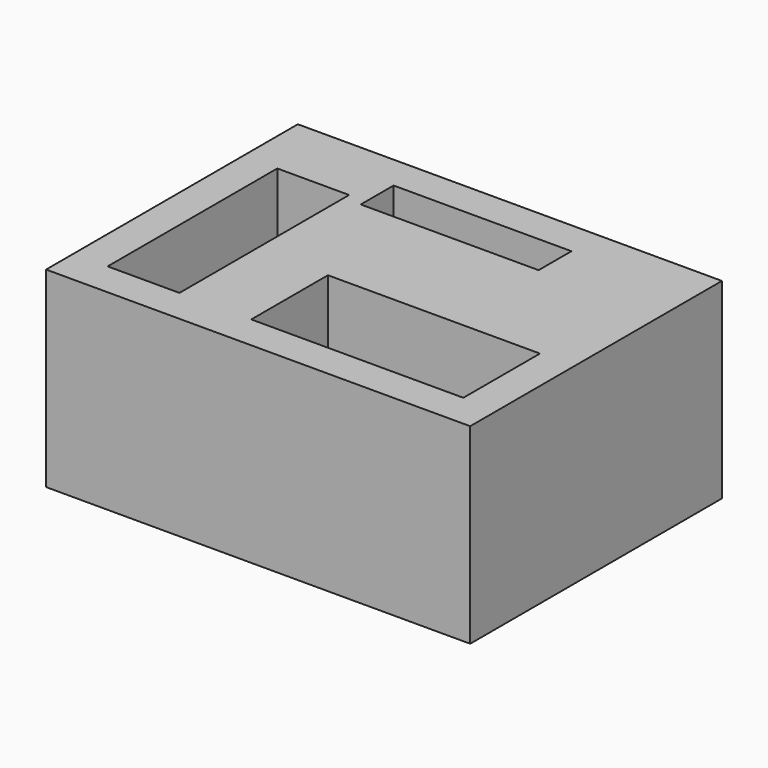
from build123d import *

# Parameters (mm, degrees)
F0_W     = 620
F0_H     = 460
F0_W_2   = 105
F0_H_2   = 310
F1_DEPTH = 280
F2_DEPTH = 250
F3_W     = 260
F3_H     = 60
F4_DEPTH = 40
F5_W     = 310
F5_H     = 140
F6_DEPTH = 155


# Not quite as in the source:
# - a feature names something its author has since deleted; it is built from what else it names


with BuildPart() as f1:
    # F0 (on Top) → F1 (new body)
    with BuildSketch(Plane.XY):
        with Locations((0.344911406, 88)):
            Rectangle(F0_W, F0_H)
        with Locations((-207.155088594, 63)):
            Rectangle(F0_W_2, F0_H_2, mode=Mode.SUBTRACT)
        with Locations((-207.155088594, 63)):
            Rectangle(F0_W_2, F0_H_2)
    extrude(amount=-F1_DEPTH)

    # F0 (on Top) → F2 (cut)
    with BuildSketch(Plane.XY):
        with Locations((-207.155088594, 63)):
            Rectangle(F0_W_2, F0_H_2)
    extrude(amount=-F2_DEPTH, mode=Mode.SUBTRACT)

    # F3 (on face) → F4 (cut)
    with BuildSketch(Plane.XY):
        with Locations((0.344911406, 238)):
            Rectangle(F3_W, F3_H)
    extrude(amount=-F4_DEPTH, mode=Mode.SUBTRACT)

    # F5 (on face) → F6 (cut)
    with BuildSketch(Plane.XY):
        with Locations((105.344911406, -22)):
            Rectangle(F5_W, F5_H)
    extrude(amount=-F6_DEPTH, mode=Mode.SUBTRACT)


solid = f1.part
